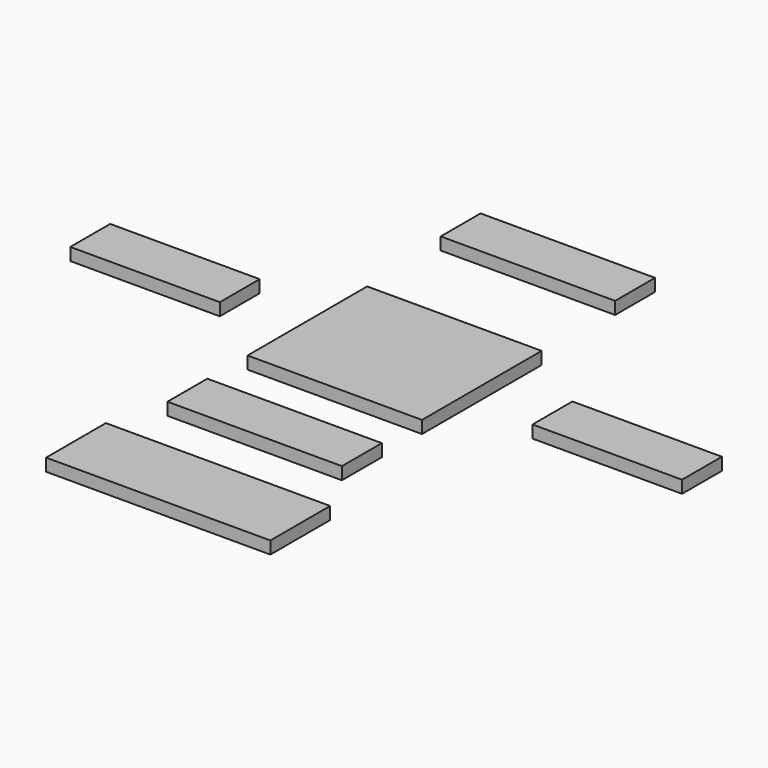
from build123d import *

# Parameters (mm, degrees)
F1_W     = 76.2
F1_H     = 25.4
F2_DEPTH = 6.35
F1_W_2   = 88.9
F1_H_2   = 76.2
F1_W_3   = 114.3
F1_H_3   = 38.1


# Not quite as in the source:
# - a variable given as a bare number and used for a length is read in inches; the dataset says mm whatever the document's units were


with BuildPart() as f2:
    # F1 (on Top) → F2 (new body)
    with BuildSketch(Plane.XY):
        with Locations((-252.0737689972, 41.6781801403)):
            Rectangle(F1_W, F1_H)
    extrude(amount=F2_DEPTH)


with BuildPart() as f2b:
    # F1 (on Top) → F2, piece 2 (new body)
    with BuildSketch(Plane.XY):
        with Locations((-132.2115360975, 38.1)):
            Rectangle(F1_W_2, F1_H_2)
    extrude(amount=F2_DEPTH)


with BuildPart() as f2c:
    # F1 (on Top) → F2, piece 3 (new body)
    with BuildSketch(Plane.XY):
        with Locations((-136.2890268325, 140.8458990288)):
            Rectangle(F1_W_2, F1_H)
    extrude(amount=F2_DEPTH)


with BuildPart() as f2d:
    # F1 (on Top) → F2, piece 4 (new body)
    with BuildSketch(Plane.XY):
        with Locations((-127.1298143625, -99.7662639737)):
            Rectangle(F1_W_3, F1_H_3)
    extrude(amount=F2_DEPTH)


with BuildPart() as f2e:
    # F1 (on Top) → F2, piece 5 (new body)
    with BuildSketch(Plane.XY):
        with Locations((-132.2115360975, -38.3136596859)):
            Rectangle(F1_W_2, F1_H)
    extrude(amount=F2_DEPTH)


with BuildPart() as f2f:
    # F1 (on Top) → F2, piece 6 (new body)
    with BuildSketch(Plane.XY):
        with Locations((-12.8600751102, 37.1072154164)):
            Rectangle(F1_W, F1_H)
    extrude(amount=F2_DEPTH)


solid = Compound([f2.part, f2b.part, f2c.part, f2d.part, f2e.part, f2f.part])
